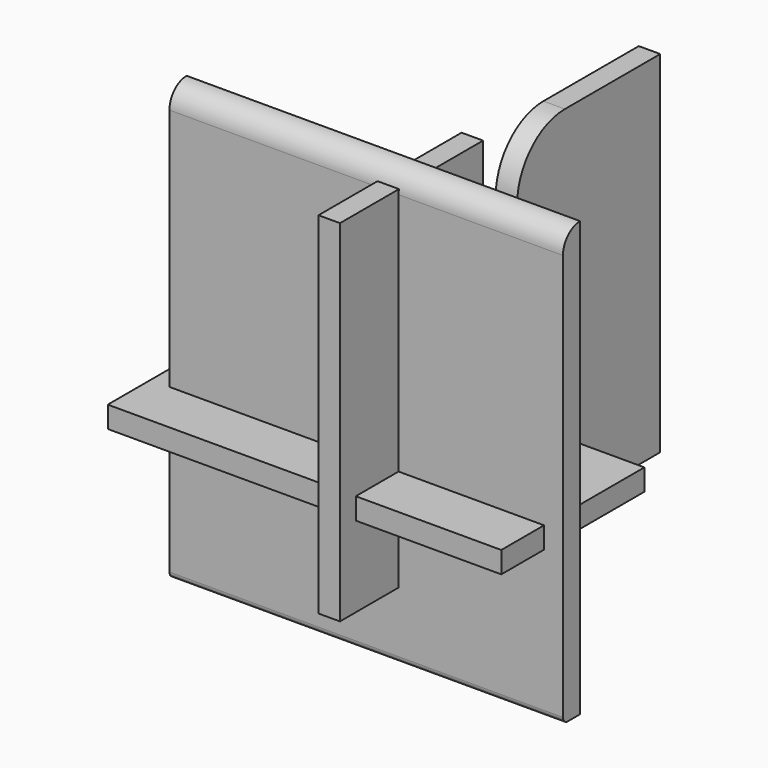
from build123d import *

# Parameters (mm, degrees)
F0_W     = 330
F0_H     = 150
F1_DEPTH = 18
F2_W     = 150
F2_H     = 294
F3_DEPTH = 18
F6_DEPTH = 18
F7_W     = 330
F7_H     = 364
F8_DEPTH = 18
F9_R     = 5
F10_R    = 17.99999


# Not quite as in the source:
# - a fillet or chamfer is up to 0.001 mm smaller than in the source, because OpenCascade refuses the exact size
# - ends of sketch curves that miss each other by under 0.0002 mm in the source are joined


with BuildPart() as f1:
    # F0 (on Top) → F1 (new body)
    with BuildSketch(Plane.XY):
        with Locations((-24.9805187998, 12.1723785996)):
            Rectangle(F0_W, F0_H)
    extrude(amount=F1_DEPTH)


with BuildPart() as f3:
    # F2 (on Right) → F3 (new body)
    with BuildSketch(Plane.YZ):
        with Locations((-4.4208914042, 79.3204397765)):
            Rectangle(F2_W, F2_H)
    extrude(amount=F3_DEPTH)


with BuildPart() as f6:
    # F5 (on face) → F6 (new body)
    with BuildSketch(Plane.YZ):
        with BuildLine():
            Line((106.3111022115, 164.7659689188), (106.3111022115, 164.7199944413))
            Line((106.3111022115, 164.7199944413), (106.3111022115, -79.2800055587))
            Line((106.3111022115, -79.2800055587), (256.3111022115, -79.2800055587))
            Line((256.3111022115, -79.2800055587), (256.3111022115, 214.7199944413))
            Line((256.3111022115, 214.7199944413), (156.3111022115, 214.7199944413))
            Line((156.3111022115, 214.7199944413), (156.3036441803, 214.7199944413))
            ThreePointArc((156.3036441803, 214.7199944413), (120.9693833899, 200.0889484934), (106.3111022115, 164.7659689188))
        make_face()
    extrude(amount=F6_DEPTH)


with BuildPart() as f8:
    # F7 (on Front) → F8 (new body)
    with BuildSketch(Plane.XZ):
        with Locations((-9.1152150415, 58.3739206195)):
            Rectangle(F7_W, F7_H)
    extrude(amount=F8_DEPTH)

    # F9
    f9_edges = [f8.edges().sort_by_distance(p)[0] for p in [
        (-9.115215, -18, -123.626079),
    ]]
    fillet(f9_edges, radius=F9_R)

    # F10 (radius 18 in the source; OpenCascade refuses exactly that, so slightly less here)
    f10_edges = [f8.edges().sort_by_distance(p)[0] for p in [
        (-9.115215, -18, 240.373921),
    ]]
    fillet(f10_edges, radius=F10_R)


solid = Compound([f1.part, f3.part, f6.part, f8.part])
